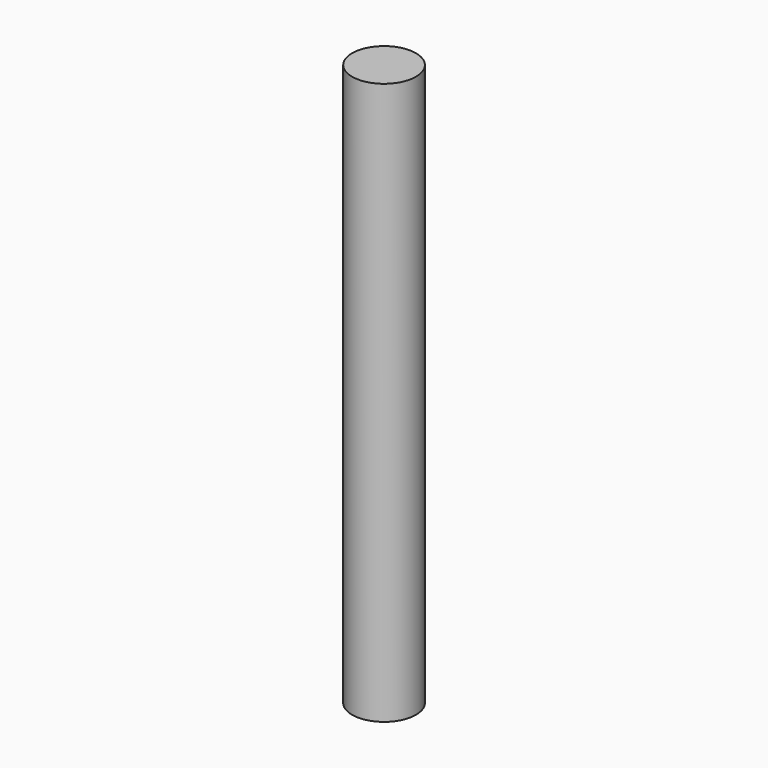
from build123d import *

# Parameters (mm, degrees)
F0_R     = 1.5875
F2_DEPTH = 27.94


# Not quite as in the source:
# - the program builds the solid bodies; features that only make, move or delete a surface that nothing else refers to are left out


with BuildPart() as f2:
    # F0 (on Top) → F2 (new body)
    with BuildSketch(Plane.XY):
        Circle(F0_R)
    extrude(amount=F2_DEPTH)


solid = f2.part
